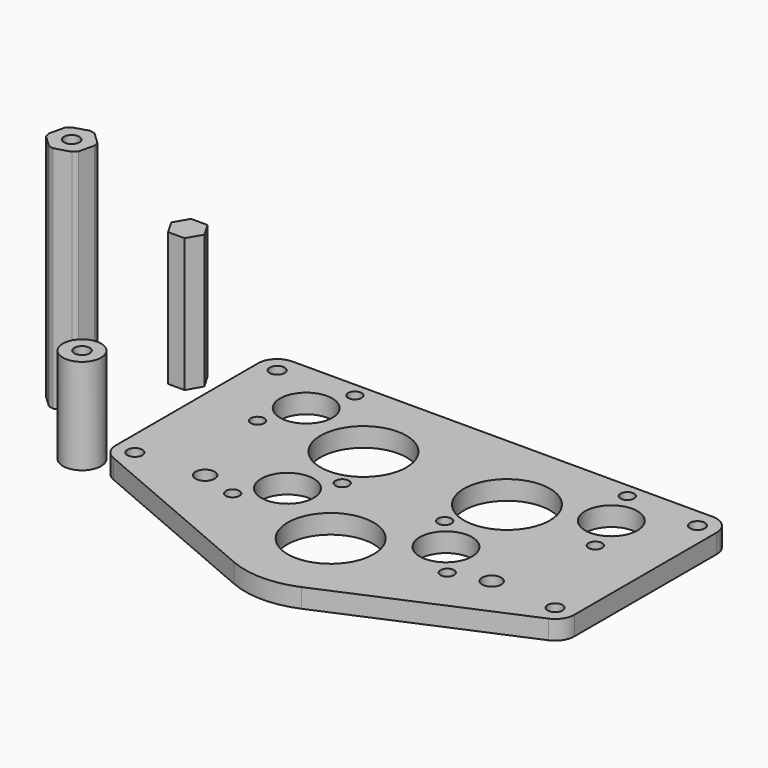
from build123d import *

# Parameters (mm, degrees)
F0_R     = 2.4892
F0_R_2   = 3.175
F0_R_3   = 2.25
F0_R_4   = 8.6995
F0_R_5   = 14.2875
F1_DEPTH = 6.35
F3_R     = 6.35
F3_R_2   = 2.54
F4_DEPTH = 31.75
F6_DEPTH = 44.45
F7_R     = 2.5527
F8_DEPTH = 76.2


# Not quite as in the source:
# - a length typed as a fraction of an inch, garbled in the dataset ("3 / 203.2 mm" for 3/8 in), is restored


with BuildPart() as f1:
    # F0 (on Top) → F1 (new body)
    with BuildSketch(Plane.XY):
        with BuildLine():
            Line((-77.202918796, 94.5181631938), (-216.902918796, 94.5181631938))
            ThreePointArc((-216.902918796, 94.5181631938), (-221.3930468565, 92.6582912543), (-223.252918796, 88.1681631938))
            Line((-223.252918796, 88.1681631938), (-223.252918796, 29.0384075017))
            ThreePointArc((-223.252918796, 29.0384075017), (-222.2047019124, 25.5436119732), (-219.4061169736, 23.2026128786))
            Line((-219.4061169736, 23.2026128786), (-158.2475012348, -3.0306844448))
            ThreePointArc((-158.2475012348, -3.0306844448), (-147.052918796, -5.3302684462), (-135.8583363571, -3.0306844448))
            Line((-135.8583363571, -3.0306844448), (-74.6997206183, 23.2026128786))
            ThreePointArc((-74.6997206183, 23.2026128786), (-71.9011356795, 25.5436119732), (-70.852918796, 29.0384075017))
            Line((-70.852918796, 29.0384075017), (-70.852918796, 88.1681631938))
            ThreePointArc((-70.852918796, 88.1681631938), (-72.7127907354, 92.6582912543), (-77.202918796, 94.5181631938))
        make_face()
        with Locations((-216.902918796, 29.0384075017)):
            Circle(F0_R, mode=Mode.SUBTRACT)
        with Locations((-194.677918796, 30.4388571531)):
            Circle(F0_R_2, mode=Mode.SUBTRACT)
        with Locations((-182.7165999633, 26.9439251239)):
            Circle(F0_R_3, mode=Mode.SUBTRACT)
        with Locations((-173.393994145, 38.0541741003)):
            Circle(F0_R_4, mode=Mode.SUBTRACT)
        with Locations((-147.052918796, 23.0676423228)):
            Circle(F0_R_5, mode=Mode.SUBTRACT)
        with Locations((-111.3892376286, 26.9439251239)):
            Circle(F0_R_3, mode=Mode.SUBTRACT)
        with Locations((-120.711843447, 38.0541741003)):
            Circle(F0_R_4, mode=Mode.SUBTRACT)
        with Locations((-99.427918796, 30.4388571531)):
            Circle(F0_R_2, mode=Mode.SUBTRACT)
        with Locations((-77.202918796, 29.0384075017)):
            Circle(F0_R, mode=Mode.SUBTRACT)
        with Locations((-203.1883047019, 62.8463448774)):
            Circle(F0_R_3, mode=Mode.SUBTRACT)
        with Locations((-164.0713883267, 49.1644230766)):
            Circle(F0_R_3, mode=Mode.SUBTRACT)
        with Locations((-170.903518796, 66.5204375982)):
            Circle(F0_R_5, mode=Mode.SUBTRACT)
        with Locations((-197.7552354349, 76.2936631938)):
            Circle(F0_R_4, mode=Mode.SUBTRACT)
        with Locations((-216.902918796, 88.1681631938)):
            Circle(F0_R, mode=Mode.SUBTRACT)
        with Locations((-192.322166168, 89.7409815101)):
            Circle(F0_R_3, mode=Mode.SUBTRACT)
        with Locations((-130.0344492653, 49.1644230766)):
            Circle(F0_R_3, mode=Mode.SUBTRACT)
        with Locations((-123.202318796, 66.5204375982)):
            Circle(F0_R_5, mode=Mode.SUBTRACT)
        with Locations((-90.9175328901, 62.8463448774)):
            Circle(F0_R_3, mode=Mode.SUBTRACT)
        with Locations((-96.350602157, 76.2936631938)):
            Circle(F0_R_4, mode=Mode.SUBTRACT)
        with Locations((-101.783671424, 89.7409815101)):
            Circle(F0_R_3, mode=Mode.SUBTRACT)
        with Locations((-77.202918796, 88.1681631938)):
            Circle(F0_R, mode=Mode.SUBTRACT)
    extrude(amount=F1_DEPTH)


with BuildPart() as f4:
    # F3 (on Top) → F4 (new body)
    with BuildSketch(Plane.XY):
        with Locations((-232.907012105, 27.0815771073)):
            Circle(F3_R)
        with Locations((-232.907012105, 27.0815771073)):
            Circle(F3_R_2, mode=Mode.SUBTRACT)
    extrude(amount=F4_DEPTH)


with BuildPart() as f6:
    # F5 (on Top) → F6 (new body)
    with BuildSketch(Plane.XY):
        Polygon((-241.8398945006, 73.9997928619), (-236.3406331865, 73.9997928619), (-233.5910025295, 78.7622928619), (-236.3406331865, 83.5247928619), (-241.8398945006, 83.5247928619), (-244.5895251576, 78.7622928619), align=None)
    extrude(amount=F6_DEPTH)


with BuildPart() as f8:
    # F7 (on Top) → F8 (new body)
    with BuildSketch(Plane.XY):
        with BuildLine():
            Line((-256.4910895061, 44.5377554726), (-251.4343531168, 46.0360276519))
            ThreePointArc((-251.4343531168, 46.0360276519), (-250.7788024003, 46.642652994), (-250.2074167827, 47.3291364414))
            Line((-250.2074167827, 47.3291364414), (-248.9765903572, 52.4575347044))
            ThreePointArc((-248.9765903572, 52.4575347044), (-249.1741679557, 53.3285709495), (-249.4829872516, 54.1666471334))
            Line((-249.4829872516, 54.1666471334), (-253.3088972154, 57.7967732171))
            ThreePointArc((-253.3088972154, 57.7967732171), (-254.1620255305, 58.06118412), (-255.042230444, 58.2127768565))
            Line((-255.042230444, 58.2127768565), (-260.0989668333, 56.7145046772))
            ThreePointArc((-260.0989668333, 56.7145046772), (-260.7545175498, 56.1078793351), (-261.3259031675, 55.4213958876))
            Line((-261.3259031675, 55.4213958876), (-262.556729593, 50.2929976246))
            ThreePointArc((-262.556729593, 50.2929976246), (-262.3591519944, 49.4219613796), (-262.0503326985, 48.5838851957))
            Line((-262.0503326985, 48.5838851957), (-258.2244227347, 44.953759112))
            ThreePointArc((-258.2244227347, 44.953759112), (-257.3712944196, 44.689348209), (-256.4910895061, 44.5377554726))
        make_face()
        with Locations((-255.7666599751, 51.3752661645)):
            Circle(F7_R, mode=Mode.SUBTRACT)
    extrude(amount=F8_DEPTH)


solid = Compound([f1.part, f4.part, f6.part, f8.part])
